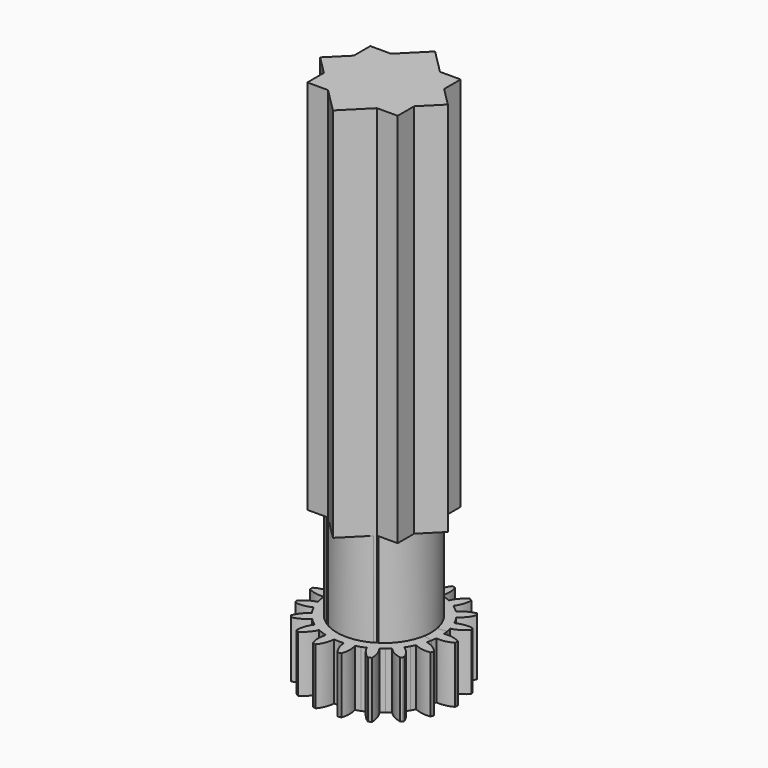
from build123d import *

# Parameters (mm, degrees)
F1_DEPTH = 3
F2_COUNT = 18
F2_ANGLE = 340
F3_DEPTH = 3
F5_DEPTH = 25
F6_R     = 5
F6_R_2   = 2.5
F7_DEPTH = 5


with BuildPart() as f1:
    # F0 (on Top) → F1 (new body)
    with BuildSketch(Plane.XY):
        with BuildLine():
            ThreePointArc((2.9885840943, 0.2614672282), (2.9743345841, 0.3915785767), (2.954423259, 0.520944533))
            Line((2.954423259, 0.520944533), (0, 0))
            Line((0, 0), (2.954423259, -0.520944533))
            ThreePointArc((2.954423259, -0.520944533), (2.9743345841, -0.3915785767), (2.9885840943, -0.2614672282))
            ThreePointArc((2.9885840943, -0.2614672282), (3.436272061, -0.2429613033), (3.8571428571, -0.0892253031))
            ThreePointArc((3.8571428571, -0.0892253031), (3.8579167462, -0.0446156348), (3.8581747207, 0))
            ThreePointArc((3.8581747207, 0), (3.8579167462, 0.0446156348), (3.8571428571, 0.0892253031))
            ThreePointArc((3.8571428571, 0.0892253031), (3.436272061, 0.2429613033), (2.9885840943, 0.2614672282))
        make_face()
    extrude(amount=F1_DEPTH)

    # F2: F1 ×18 about axis
    f2_axis = Axis((0, 0, 1.5), (0, 0, -1))


with BuildPart() as f1_1:
    add(f1.part)
    for i in range(1, F2_COUNT):
        add(f1.part.rotate(f2_axis, i * F2_ANGLE / (F2_COUNT - 1)))

    # F4 (on face) → F5 (join)
    with BuildSketch(Plane.XY.offset(3)):
        Polygon((1.3019114351, -2.0922011145), (2.4, -2.0922011145), (2.4, -0.9941125497), align=None)
        Polygon((0, -3.3941125497), (1.3019114351, -2.0922011145), (-1.3019114351, -2.0922011145), align=None)
        Polygon((-1.3019114351, -2.0922011145), (1.3019114351, -2.0922011145), (2.4, -0.9941125497), (2.4, 0.9941125497), (1.3019114351, 2.0922011145), (-1.3019114351, 2.0922011145), (-2.4, 0.9941125497), (-2.4, -0.9941125497), align=None)
        Polygon((2.4, 0.9941125497), (2.4, -0.9941125497), (3.3941125497, 0), align=None)
        Polygon((-2.4, -2.0922011145), (-1.3019114351, -2.0922011145), (-2.4, -0.9941125497), align=None)
        Polygon((1.3019114351, 2.0922011145), (2.4, 0.9941125497), (2.4, 2.0922011145), align=None)
        Polygon((-3.3941125497, 0), (-2.4, -0.9941125497), (-2.4, 0.9941125497), align=None)
        Polygon((-1.3019114351, 2.0922011145), (1.3019114351, 2.0922011145), (0, 3.3941125497), align=None)
        Polygon((-2.4, 2.0922011145), (-2.4, 0.9941125497), (-1.3019114351, 2.0922011145), align=None)
    extrude(amount=F5_DEPTH)

    # F6 (on face) → F7 (cut)
    with BuildSketch(Plane.XY.offset(3)):
        Circle(F6_R)
        Circle(F6_R_2, mode=Mode.SUBTRACT)
    extrude(amount=F7_DEPTH, mode=Mode.SUBTRACT)


with BuildPart() as f3:
    # F0 (on Top) → F3 (new body)
    with BuildSketch(Plane.XY):
        with BuildLine():
            ThreePointArc((2.9885840943, 0.2614672282), (2.9743345841, 0.3915785767), (2.954423259, 0.520944533))
            Line((2.954423259, 0.520944533), (0, 0))
            Line((0, 0), (2.954423259, -0.520944533))
            ThreePointArc((2.954423259, -0.520944533), (2.9743345841, -0.3915785767), (2.9885840943, -0.2614672282))
            ThreePointArc((2.9885840943, -0.2614672282), (3.436272061, -0.2429613033), (3.8571428571, -0.0892253031))
            ThreePointArc((3.8571428571, -0.0892253031), (3.8579167462, -0.0446156348), (3.8581747207, 0))
            ThreePointArc((3.8581747207, 0), (3.8579167462, 0.0446156348), (3.8571428571, 0.0892253031))
            ThreePointArc((3.8571428571, 0.0892253031), (3.436272061, 0.2429613033), (2.9885840943, 0.2614672282))
        make_face()
    extrude(amount=F3_DEPTH)


solid = Compound([f1_1.part, f3.part])
